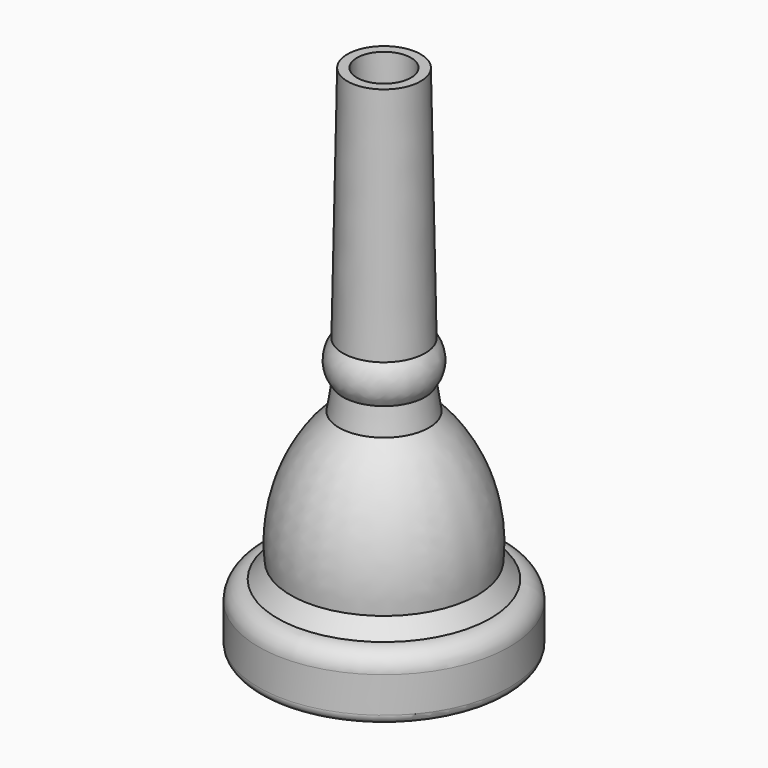
from build123d import *

# Parameters (mm, degrees)
F3_R = 1.5
F4_R = 5


# Not quite as in the source:
# - a fillet or chamfer that OpenCascade refuses, or shapes differently, is made with other operations: its cross-section is extruded or revolved along the edge and cut away or added


with BuildPart() as f1:
    # F0 (on Front) → F1 (revolve)
    with BuildSketch(Plane.XZ):
        with BuildLine():
            Line((-3.2761832158, -65.334129345), (-5.337398374, -62.834129345))
            ThreePointArc((-5.337398374, -62.834129345), (-6.7311516997, -51.7224852161), (-12.8360642807, -42.334129345))
            Line((-12.8360642807, -42.334129345), (-13.4396579748, -38.334129345))
            ThreePointArc((-13.4396579748, -38.334129345), (-12.3713927582, -35.334129345), (-13.4396579748, -32.334129345))
            Line((-13.4396579748, -32.334129345), (-14.137398374, 4.665870655))
            Line((-14.137398374, 4.665870655), (-15.637398374, 4.665870655))
            Line((-15.637398374, 4.665870655), (-16.837398374, -50.334129345))
            ThreePointArc((-16.837398374, -50.334129345), (-9.9295742391, -59.4637716742), (-6.337398374, -70.334129345))
            Line((-6.337398374, -70.334129345), (-6.337398374, -75.334129345))
            Line((-6.337398374, -75.334129345), (-0.337398374, -75.334129345))
            Line((-0.337398374, -75.334129345), (-0.337398374, -65.334129345))
            Line((-0.337398374, -65.334129345), (-3.2761832158, -65.334129345))
        make_face()
    revolve(axis=Axis((-19.837398374, 0, -35.334129345), (0, 0, 1)))

    # F2: fillet of radius 3 on 1 edges, made by hand

    # F2_s1 → F2_t2 (revolve, cut)
    with BuildSketch(Plane.XZ):
        with BuildLine():
            ThreePointArc((-0.336998374, -68.3344507591), (-1.1942035822, -66.2342669991), (-3.2761749277, -65.3337294309))
            Line((-3.2761749277, -65.3337294309), (-3.2699560145, -65.0336572981))
            ThreePointArc((-3.2699560145, -65.0336572981), (-1.8067866508, -65.0339927765), (-0.337398374, -65.0339927765))
            Line((-0.337398374, -65.0339927765), (-0.0372618054, -65.334129345))
            ThreePointArc((-0.0372618054, -65.334129345), (-0.0372618054, -66.8342900521), (-0.0368618054, -68.3344507591))
            Line((-0.0368618054, -68.3344507591), (-0.336998374, -68.3344507591))
        make_face()
    revolve(axis=Axis((-19.837398374, 0, -65.334129345), (0, 0, 1)), mode=Mode.SUBTRACT)

    # F3
    f3_edges = [f1.edges().sort_by_distance(p)[0] for p in [
        (-33.337398, 0, -75.334129),
        (-39.337398, 0, -75.334129),
    ]]
    fillet(f3_edges, radius=F3_R)

    # F4
    f4_edges = [f1.edges().sort_by_distance(p)[0] for p in [
        (-22.837398, 0, -50.334129),
    ]]
    fillet(f4_edges, radius=F4_R)


solid = f1.part
